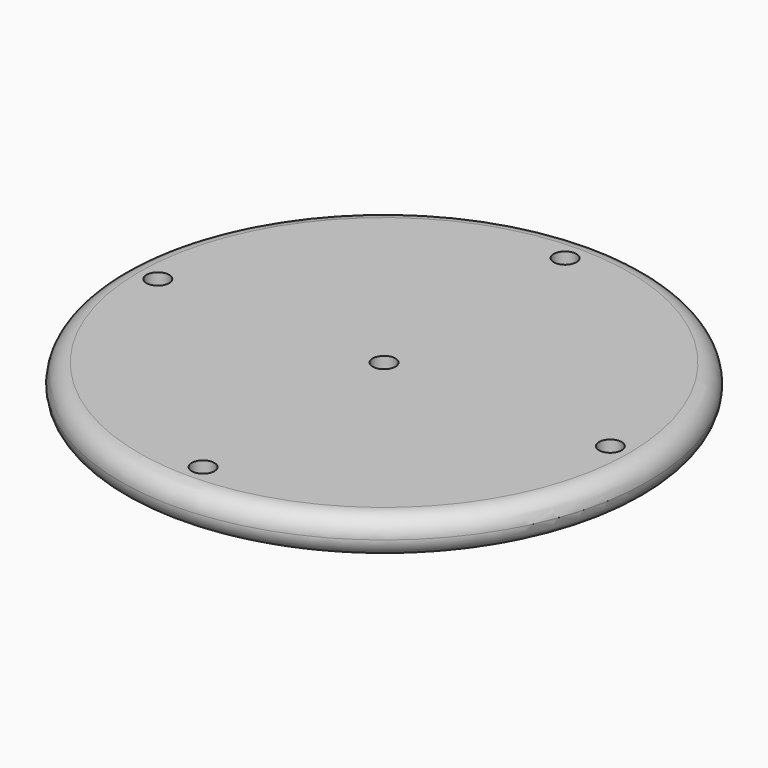
from build123d import *

# Parameters (mm, degrees)
F0_R     = 35
F0_R_2   = 1.5
F1_DEPTH = 5
F2_R     = 2.49999
F3_D     = 3


# Not quite as in the source:
# - a fillet or chamfer is up to 0.001 mm smaller than in the source, because OpenCascade refuses the exact size


with BuildPart() as f1:
    # F0 (on Top) → F1 (new body)
    with BuildSketch(Plane.XY):
        Circle(F0_R)
        with Locations((0, -30)):
            Circle(F0_R_2, mode=Mode.SUBTRACT)
        with Locations((-30, 0)):
            Circle(F0_R_2, mode=Mode.SUBTRACT)
        with Locations((30, 0)):
            Circle(F0_R_2, mode=Mode.SUBTRACT)
        with Locations((0, 30)):
            Circle(F0_R_2, mode=Mode.SUBTRACT)
    extrude(amount=F1_DEPTH)

    # F2 (radius 2.5 in the source; OpenCascade refuses exactly that, so slightly less here)
    f2_edges = [f1.edges().sort_by_distance(p)[0] for p in [
        (-35, 0, 5),
        (-35, 0, 0),
    ]]
    fillet(f2_edges, radius=F2_R)

    # F3 (through all)
    with Locations(Plane(origin=(0, 0, 0), x_dir=(1, 0, 0), z_dir=(0, 0, -1))):
        with Locations((0, 0)):
            Hole(F3_D / 2)


solid = f1.part
